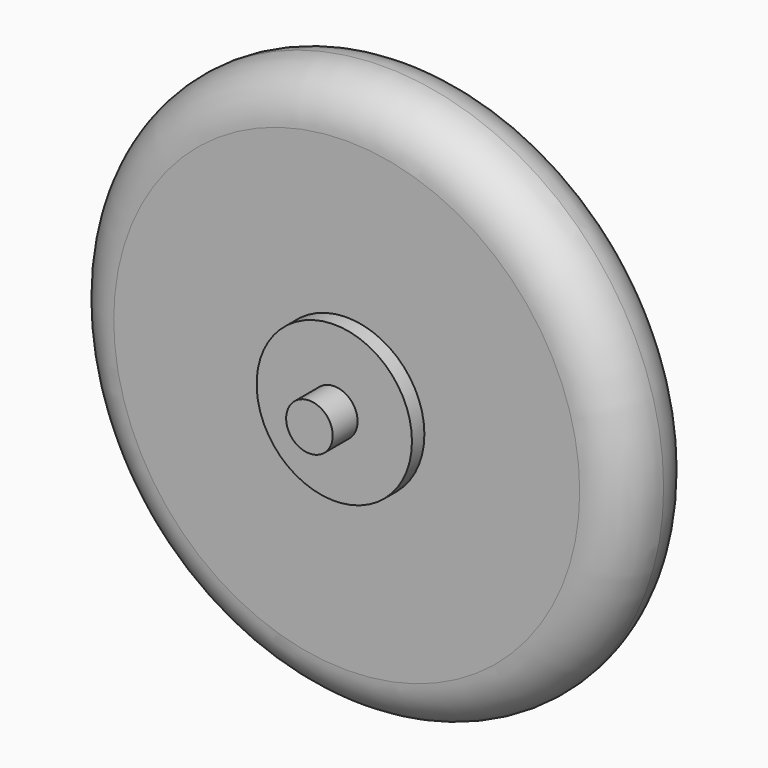
from build123d import *

# Parameters (mm, degrees)
F0_R          = 90
F0_R_2        = 25
F1_DEPTH      = 30
F0_R_3        = 7.5
F2_DEPTH      = 35
F3_R          = 14.99999
F4_DEPTH      = 5
F5_DEPTH      = 15
F5_DEPTH_BACK = 45


# Not quite as in the source:
# - a fillet or chamfer is up to 0.001 mm smaller than in the source, because OpenCascade refuses the exact size


with BuildPart() as f1:
    # F0 (on Front) → F1 (new body)
    with BuildSketch(Plane.XZ):
        Circle(F0_R)
        Circle(F0_R_2, mode=Mode.SUBTRACT)
    extrude(amount=F1_DEPTH)

    # F0 (on Front) → F2 (join)
    with BuildSketch(Plane.XZ):
        Circle(F0_R_2)
        Circle(F0_R_3, mode=Mode.SUBTRACT)
    extrude(amount=F2_DEPTH)

    # F3 (radius 15 in the source; OpenCascade refuses exactly that, so slightly less here)
    f3_edges = [f1.edges().sort_by_distance(p)[0] for p in [
        (-90, -30, 0),
        (-90, 0, 0),
    ]]
    fillet(f3_edges, radius=F3_R)

    # F0 (on Front) → F4 (join)
    with BuildSketch(Plane.XZ):
        Circle(F0_R_2)
        Circle(F0_R_3, mode=Mode.SUBTRACT)
    extrude(amount=-F4_DEPTH)

    # F0 (on Front) → F5 (join, two sides)
    with BuildSketch(Plane.XZ) as f5_sk:
        Circle(F0_R_3)
    extrude(amount=-F5_DEPTH)
    extrude(f5_sk.sketch, amount=F5_DEPTH_BACK)


solid = f1.part
